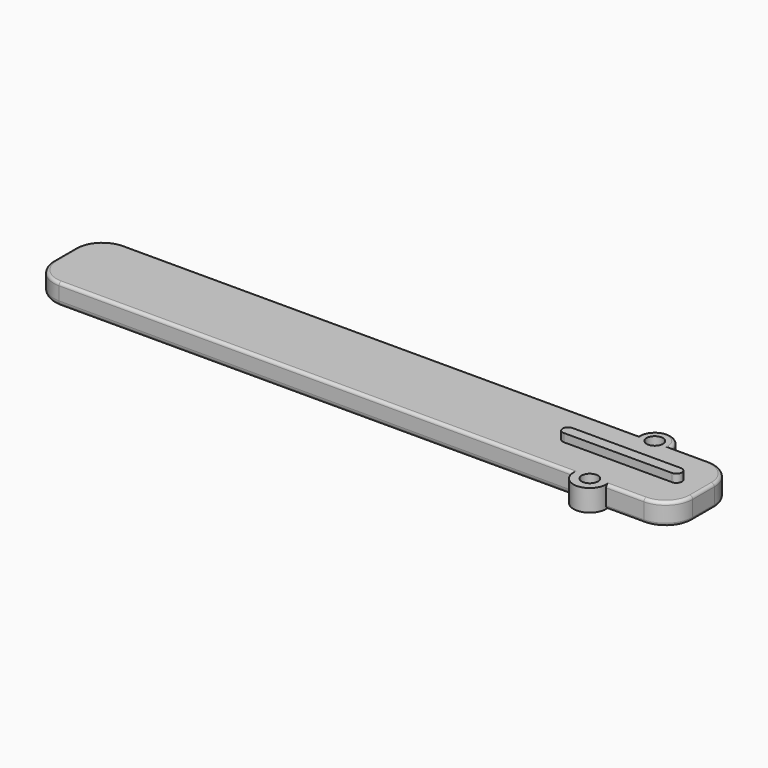
from build123d import *
from build123d import SkipClean  # not in build123d's __all__

# Parameters (mm, degrees)
F0_R     = 1.5
F1_DEPTH = 4
F2_R     = 0.55
F3_R     = 1
F4_R     = 0.5499
F6_DEPTH = 5.5


# Not quite as in the source:
# - a fillet or chamfer is up to 0.001 mm smaller than in the source, because OpenCascade refuses the exact size
# - a feature names something its author has since deleted; it is built from what else it names


with BuildPart() as f1:
    # F0 (on Top) → F1 (new body)
    with BuildSketch(Plane.XY):
        with BuildLine():
            Line((-95, 0), (0, 0))
            ThreePointArc((0, 0), (3, -3), (6, 0))
            Line((6, 0), (13, 0))
            ThreePointArc((13, 0), (16.5355339059, 1.4644660941), (18, 5))
            Line((18, 5), (18, 10))
            ThreePointArc((18, 10), (16.5355339059, 13.5355339059), (13, 15))
            Line((13, 15), (6, 15))
            ThreePointArc((6, 15), (3, 18), (0, 15))
            Line((0, 15), (-95, 15))
            ThreePointArc((-95, 15), (-98.5355339059, 13.5355339059), (-100, 10))
            Line((-100, 10), (-100, 5))
            ThreePointArc((-100, 5), (-98.5355339059, 1.4644660941), (-95, 0))
        make_face()
        with Locations((3, 0)):
            Circle(F0_R, mode=Mode.SUBTRACT)
        with Locations((3, 15)):
            Circle(F0_R, mode=Mode.SUBTRACT)
    extrude(amount=F1_DEPTH)

    # F2
    f2_edges = [f1.edges().sort_by_distance(p)[0] for p in [
        (-47.5, 0, 4),
    ]]
    fillet(f2_edges, radius=F2_R)

    # F3
    f3_edges = [f1.edges().sort_by_distance(p)[0] for p in [
        (-47.5, 0, 0),
    ]]
    fillet(f3_edges, radius=F3_R)

    # F4 (radius 0.55 in the source; OpenCascade refuses exactly that, so slightly less here)
    f4_edges = [f1.edges().sort_by_distance(p)[0] for p in [
        (3, 18, 4),
        (3, 18, 0),
        (9.5, 0, 4),
        (16.535534, 13.535534, 4),
        (16.535534, 1.464466, 4),
        (16.535534, 13.535534, 0),
        (16.535534, 1.464466, 0),
        (9.5, 0, 0),
        (9.5, 15, 0),
        (9.5, 15, 4),
    ]]
    fillet(f4_edges, radius=F4_R)

    # F5 (on Top) → F6 (join)
    with BuildSketch(Plane.XY):
        with BuildLine():
            Line((12.9997539334, 8.5000049546), (-6.9997087121, 8.5000049546))
            ThreePointArc((-6.9997087121, 8.5000049546), (-7.9997087121, 7.5000049546), (-6.9997087121, 6.5000049546))
            Line((-6.9997087121, 6.5000049546), (12.9997539334, 6.5000049546))
            ThreePointArc((12.9997539334, 6.5000049546), (13.9997539334, 7.5000049546), (12.9997539334, 8.5000049546))
        make_face()
    with SkipClean():  # cleaning this boolean's faces spoils the solid; the shape is the same uncleaned
        extrude(amount=F6_DEPTH)


solid = f1.part
